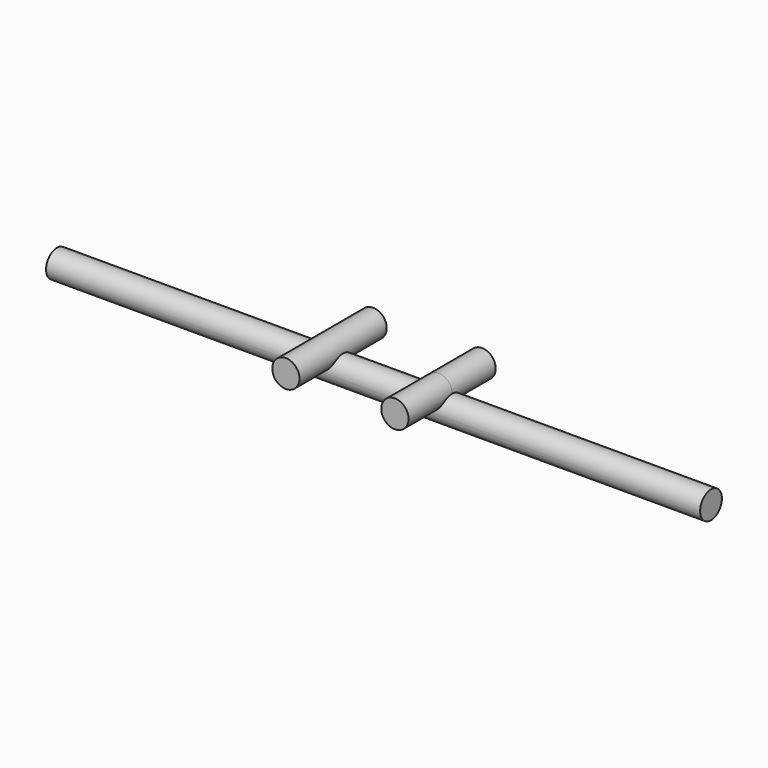
from build123d import *

# Parameters (mm, degrees)
F0_R     = 3.175
F1_DEPTH = 152.4
F2_R     = 3.175
F3_DEPTH = 12.7


# Not quite as in the source:
# - a feature names something its author has since deleted; it is built from what else it names


with BuildPart() as f1:
    # F0 (on Right) → F1 (new body)
    with BuildSketch(Plane.YZ):
        with Locations((0, -3.175)):
            Circle(F0_R)
    extrude(amount=F1_DEPTH)

    # F2 (on Front) → F3 (join, symmetric)
    with BuildSketch(Plane.XZ):
        with BuildLine():
            ThreePointArc((92.075, 0), (88.9, 3.175), (85.725, 0))
            ThreePointArc((85.725, 0), (88.9, -3.175), (92.075, 0))
        make_face()
        with Locations((63.5, 0)):
            Circle(F2_R)
    extrude(amount=F3_DEPTH, both=True)


solid = f1.part
